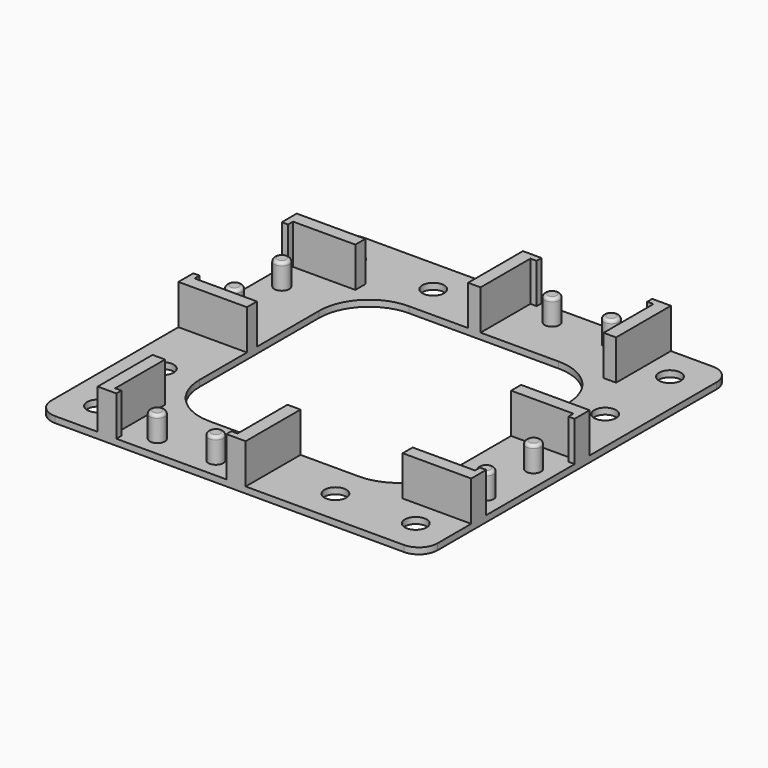
from build123d import *

# Parameters (mm, degrees)
F1_DEPTH    = 7.4
F0_R        = 1.2
F2_DEPTH    = 5
F0_R_2      = 1.75
F3_DEPTH    = 1
F4_R        = 3
F5_R        = 0.5
F6_T1_DEPTH = 1


# Not quite as in the source:
# - a fillet or chamfer that OpenCascade refuses, or shapes differently, is made with other operations: its cross-section is extruded or revolved along the edge and cut away or added


with BuildPart() as f1:
    # F0 (on Top) → F1 (new body)
    with BuildSketch(Plane.XY):
        Polygon((-2.5, 20), (-0.5, 20), (-0.5, 30), (0.5, 30), (0.5, 31), (0, 31), (-2.5, 31), align=None)
    extrude(amount=F1_DEPTH)



with BuildPart() as f1b:
    # F0 (on Top) → F1, piece 2 (new body)
    with BuildSketch(Plane.XY):
        Polygon((19.25, 30), (19.25, 20), (20, 20), (21.25, 20), (21.25, 31), (18.25, 31), (18.25, 30), align=None)
    extrude(amount=F1_DEPTH)


with BuildPart() as f1c:
    # F0 (on Top) → F1, piece 3 (new body)
    with BuildSketch(Plane.XY):
        Polygon((31, 2.5), (20, 2.5), (20, 0.5), (30, 0.5), (30, -0.5), (31, -0.5), align=None)
    extrude(amount=F1_DEPTH)


with BuildPart() as f1d:
    # F0 (on Top) → F1, piece 4 (new body)
    with BuildSketch(Plane.XY):
        Polygon((30, -19.25), (20, -19.25), (20, -20), (20, -21.25), (31, -21.25), (31, -18.25), (30, -18.25), align=None)
    extrude(amount=F1_DEPTH)


with BuildPart() as f1e:
    # F0 (on Top) → F1, piece 5 (new body)
    with BuildSketch(Plane.XY):
        Polygon((2.599675854, -31), (2.599675854, -20), (0.5, -20), (0.5, -30), (-0.5, -30), (-0.5, -31), (0, -31), align=None)
    extrude(amount=F1_DEPTH)


with BuildPart() as f1f:
    # F0 (on Top) → F1, piece 6 (new body)
    with BuildSketch(Plane.XY):
        Polygon((-19.150324146, -20), (-20, -20), (-21.150324146, -20), (-21.150324146, -31), (-18.150324146, -31), (-18.150324146, -30), (-19.150324146, -30), align=None)
    extrude(amount=F1_DEPTH)


with BuildPart() as f1g:
    # F0 (on Top) → F1, piece 7 (new body)
    with BuildSketch(Plane.XY):
        Polygon((-20, -2.5), (-20, -0.5), (-30, -0.5), (-30, 0.5), (-31, 0.5), (-31, -2.5), align=None)
    extrude(amount=F1_DEPTH)


with BuildPart() as f1h:
    # F0 (on Top) → F1, piece 8 (new body)
    with BuildSketch(Plane.XY):
        Polygon((-20, 19.25), (-20, 20), (-20, 21.25), (-31, 21.25), (-31, 18.25), (-30, 18.25), (-30, 19.25), align=None)
    extrude(amount=F1_DEPTH)


with BuildPart() as f2:
    # F0 (on Top) → F2 (new body)
    with BuildSketch(Plane.XY):
        with Locations((4.75, 27.8)):
            Circle(F0_R)
    extrude(amount=F2_DEPTH)


with BuildPart() as f2b:
    # F0 (on Top) → F2, piece 2 (new body)
    with BuildSketch(Plane.XY):
        with Locations((14.25, 27.8)):
            Circle(F0_R)
    extrude(amount=F2_DEPTH)


with BuildPart() as f2c:
    # F0 (on Top) → F2, piece 3 (new body)
    with BuildSketch(Plane.XY):
        with Locations((27.8, -4.75)):
            Circle(F0_R)
    extrude(amount=F2_DEPTH)


with BuildPart() as f2d:
    # F0 (on Top) → F2, piece 4 (new body)
    with BuildSketch(Plane.XY):
        with Locations((27.8, -14.25)):
            Circle(F0_R)
    extrude(amount=F2_DEPTH)


with BuildPart() as f2e:
    # F0 (on Top) → F2, piece 5 (new body)
    with BuildSketch(Plane.XY):
        with Locations((-4.75, -27.8)):
            Circle(F0_R)
    extrude(amount=F2_DEPTH)


with BuildPart() as f2f:
    # F0 (on Top) → F2, piece 6 (new body)
    with BuildSketch(Plane.XY):
        with Locations((-14.150324146, -27.8)):
            Circle(F0_R)
    extrude(amount=F2_DEPTH)


with BuildPart() as f2g:
    # F0 (on Top) → F2, piece 7 (new body)
    with BuildSketch(Plane.XY):
        with Locations((-27.8, 14.25)):
            Circle(F0_R)
    extrude(amount=F2_DEPTH)


with BuildPart() as f2h:
    # F0 (on Top) → F2, piece 8 (new body)
    with BuildSketch(Plane.XY):
        with Locations((-27.8, 4.75)):
            Circle(F0_R)
    extrude(amount=F2_DEPTH)


with BuildPart() as f1_1:
    add(f1.part)

    add(f1b.part)  # F3 merges F1b

    add(f1c.part)  # F3 merges F1c

    add(f1d.part)  # F3 merges F1d

    add(f1e.part)  # F3 merges F1e

    add(f1f.part)  # F3 merges F1f

    add(f1g.part)  # F3 merges F1g

    add(f1h.part)  # F3 merges F1h

    add(f2.part)  # F3 merges F2

    add(f2b.part)  # F3 merges F2b

    add(f2c.part)  # F3 merges F2c

    add(f2d.part)  # F3 merges F2d

    add(f2e.part)  # F3 merges F2e

    add(f2f.part)  # F3 merges F2f

    add(f2g.part)  # F3 merges F2g

    add(f2h.part)  # F3 merges F2h
    # F0 (on Top) → F3 (join)
    with BuildSketch(Plane.XY):
        Polygon((-0.5, 20), (0, 20), (19.25, 20), (19.25, 30), (18.25, 30), (18.25, 31), (0.5, 31), (0.5, 30), (-0.5, 30), align=None)
        with Locations((4.75, 27.8)):
            Circle(F0_R, mode=Mode.SUBTRACT)
        with Locations((14.25, 27.8)):
            Circle(F0_R, mode=Mode.SUBTRACT)
        Polygon((-20, 20), (-2.5, 20), (-2.5, 31), (-31, 31), (-31, 21.25), (-20, 21.25), align=None)
        with Locations((-25.5, 25.5)):
            Circle(F0_R_2, mode=Mode.SUBTRACT)
        with Locations((-12.5, 25.5)):
            Circle(F0_R_2, mode=Mode.SUBTRACT)
        Polygon((-20, -0.5), (-20, 19.25), (-30, 19.25), (-30, 18.25), (-31, 18.25), (-31, 0.5), (-30, 0.5), (-30, -0.5), align=None)
        with Locations((-27.8, 4.75)):
            Circle(F0_R, mode=Mode.SUBTRACT)
        with Locations((-27.8, 14.25)):
            Circle(F0_R, mode=Mode.SUBTRACT)
        Polygon((-20, -20), (-20, -2.5), (-31, -2.5), (-31, -31), (-21.150324146, -31), (-21.150324146, -20), align=None)
        with Locations((-25.5, -25.5)):
            Circle(F0_R_2, mode=Mode.SUBTRACT)
        with Locations((-25.5, -12.5)):
            Circle(F0_R_2, mode=Mode.SUBTRACT)
        Polygon((0.5, -30), (0.5, -20), (0, -20), (-17.1610249381, -20), (-19.150324146, -20), (-19.150324146, -30), (-18.150324146, -30), (-18.150324146, -31), (-17.1610249381, -31), (-3.6785447102, -31), (-0.5, -31), (-0.5, -30), align=None)
        with Locations((-14.150324146, -27.8)):
            Circle(F0_R, mode=Mode.SUBTRACT)
        with Locations((-4.75, -27.8)):
            Circle(F0_R, mode=Mode.SUBTRACT)
        Polygon((20, -21.25), (20, -20), (2.599675854, -20), (2.599675854, -31), (31, -31), (31, -21.25), align=None)
        with Locations((12.599675854, -25.5)):
            Circle(F0_R_2, mode=Mode.SUBTRACT)
        with Locations((25.5, -25.5)):
            Circle(F0_R_2, mode=Mode.SUBTRACT)
        Polygon((30, 0.5), (20, 0.5), (20, -19.25), (30, -19.25), (30, -18.25), (31, -18.25), (31, -0.5), (30, -0.5), align=None)
        with Locations((27.8, -14.25)):
            Circle(F0_R, mode=Mode.SUBTRACT)
        with Locations((27.8, -4.75)):
            Circle(F0_R, mode=Mode.SUBTRACT)
        Polygon((21.25, 20), (20, 20), (20, 2.5), (31, 2.5), (31, 31), (21.25, 31), align=None)
        with Locations((25.5, 12.5)):
            Circle(F0_R_2, mode=Mode.SUBTRACT)
        with Locations((25.5, 25.5)):
            Circle(F0_R_2, mode=Mode.SUBTRACT)
    extrude(amount=F3_DEPTH)

    # F4
    f4_edges = [f1_1.edges().sort_by_distance(p)[0] for p in [
        (-31, 31, 0.5),
        (31, 31, 0.5),
        (31, -31, 0.5),
        (-31, -31, 0.5),
    ]]
    fillet(f4_edges, radius=F4_R)

    # F5
    f5_edges = [f1_1.edges().sort_by_distance(p)[0] for p in [
        (13.05, 27.8, 5),
        (3.55, 27.8, 5),
        (-29, 14.25, 5),
        (-29, 4.75, 5),
        (26.6, -4.75, 5),
        (26.6, -14.25, 5),
        (-5.95, -27.8, 5),
        (-15.350324, -27.8, 5),
    ]]
    fillet(f5_edges, radius=F5_R)

    # F6: fillet of radius 8 on 4 edges, made by hand

    # F6_s2 → F6_t1 (join)
    with BuildSketch(Plane.XY):
        with BuildLine():
            ThreePointArc((-20, -12), (-17.6568542495, -17.6568542495), (-12, -20))
            Line((-12, -20), (-20, -20))
            Line((-20, -20), (-20, -12))
        make_face()
        with BuildLine():
            ThreePointArc((12, -20), (17.6568542495, -17.6568542495), (20, -12))
            Line((20, -12), (20, -20))
            Line((20, -20), (12, -20))
        make_face()
        with BuildLine():
            ThreePointArc((12, 20), (17.6568542495, 17.6568542495), (20, 12))
            Line((20, 12), (20, 20))
            Line((20, 20), (12, 20))
        make_face()
        with BuildLine():
            ThreePointArc((-20, 12), (-17.6568542495, 17.6568542495), (-12, 20))
            Line((-12, 20), (-20, 20))
            Line((-20, 20), (-20, 12))
        make_face()
    extrude(amount=F6_T1_DEPTH)


solid = f1_1.part
